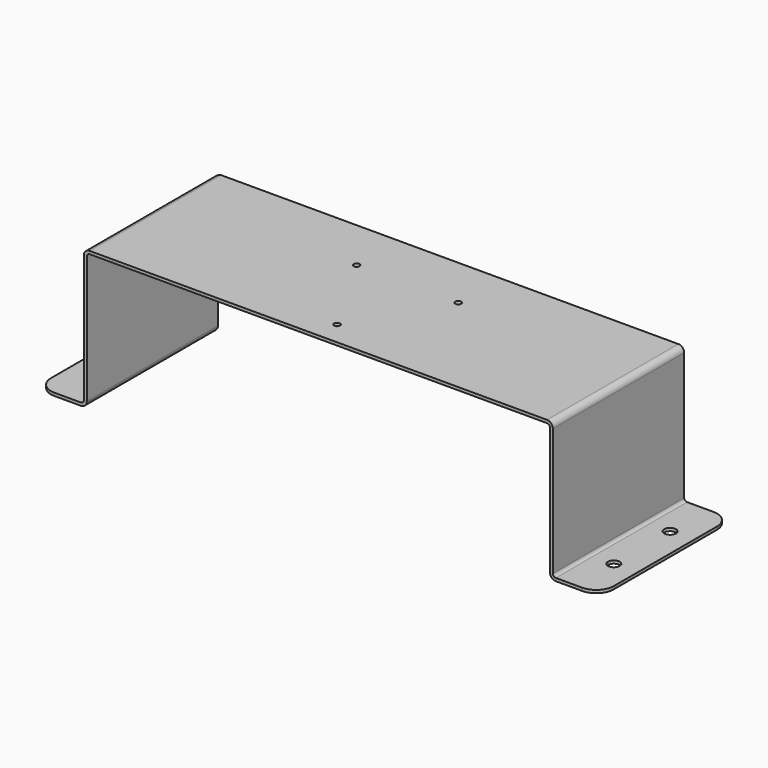
from build123d import *

# Parameters (mm, degrees)
F1_DEPTH = 44.45
F2_R     = 3.175
F2_R_2   = 1.5875
F3_DEPTH = 75.40725
F4_R     = 9.525


with BuildPart() as f1:
    # F0 (on Front) → F1 (new body, symmetric)
    with BuildSketch(Plane.XZ):
        with BuildLine():
            Line((-125.4125, 0), (-1.5875, 0))
            ThreePointArc((-1.5875, 0), (-0.4649679849, -0.4649679849), (0, -1.5875))
            Line((0, -1.5875), (0, -70.64375))
            ThreePointArc((0, -70.64375), (0.9299359697, -72.8888140303), (3.175, -73.81875))
            Line((3.175, -73.81875), (26.9875, -73.81875))
            Line((26.9875, -73.81875), (26.9875, -72.23125))
            Line((26.9875, -72.23125), (3.175, -72.23125))
            ThreePointArc((3.175, -72.23125), (2.0524679849, -71.7662820151), (1.5875, -70.64375))
            Line((1.5875, -70.64375), (1.5875, -1.5875))
            ThreePointArc((1.5875, -1.5875), (0.6575640303, 0.6575640303), (-1.5875, 1.5875))
            Line((-1.5875, 1.5875), (-125.4125, 1.5875))
            Line((-125.4125, 1.5875), (-249.2375, 1.5875))
            ThreePointArc((-249.2375, 1.5875), (-251.4825640303, 0.6575640303), (-252.4125, -1.5875))
            Line((-252.4125, -1.5875), (-252.4125, -70.64375))
            ThreePointArc((-252.4125, -70.64375), (-252.8774679849, -71.7662820151), (-254, -72.23125))
            Line((-254, -72.23125), (-277.8125, -72.23125))
            Line((-277.8125, -72.23125), (-277.8125, -73.81875))
            Line((-277.8125, -73.81875), (-254, -73.81875))
            ThreePointArc((-254, -73.81875), (-251.7549359697, -72.8888140303), (-250.825, -70.64375))
            Line((-250.825, -70.64375), (-250.825, -1.5875))
            ThreePointArc((-250.825, -1.5875), (-250.3600320151, -0.4649679849), (-249.2375, 0))
            Line((-249.2375, 0), (-125.4125, 0))
        make_face()
    extrude(amount=F1_DEPTH, both=True)

    # F2 (on face) → F3 (cut, through all)
    with BuildSketch(Plane.XY.offset(1.5875)):
        with Locations((14.2875, 19.05)):
            Circle(F2_R)
        with Locations((14.2875, -19.05)):
            Circle(F2_R)
        with Locations((-125.4125, -31.75)):
            Circle(F2_R_2)
        with Locations((-97.9161934298, 15.875)):
            Circle(F2_R_2)
        with Locations((-152.9088065702, 15.875)):
            Circle(F2_R_2)
        with Locations((-265.1125, 19.05)):
            Circle(F2_R)
        with Locations((-265.1125, -19.05)):
            Circle(F2_R)
    extrude(amount=-F3_DEPTH, mode=Mode.SUBTRACT)

    # F4
    f4_edges = [f1.edges().sort_by_distance(p)[0] for p in [
        (26.9875, 44.45, -73.025),
        (26.9875, -44.45, -73.025),
        (-277.8125, -44.45, -73.025),
        (-277.8125, 44.45, -73.025),
    ]]
    fillet(f4_edges, radius=F4_R)


solid = f1.part
